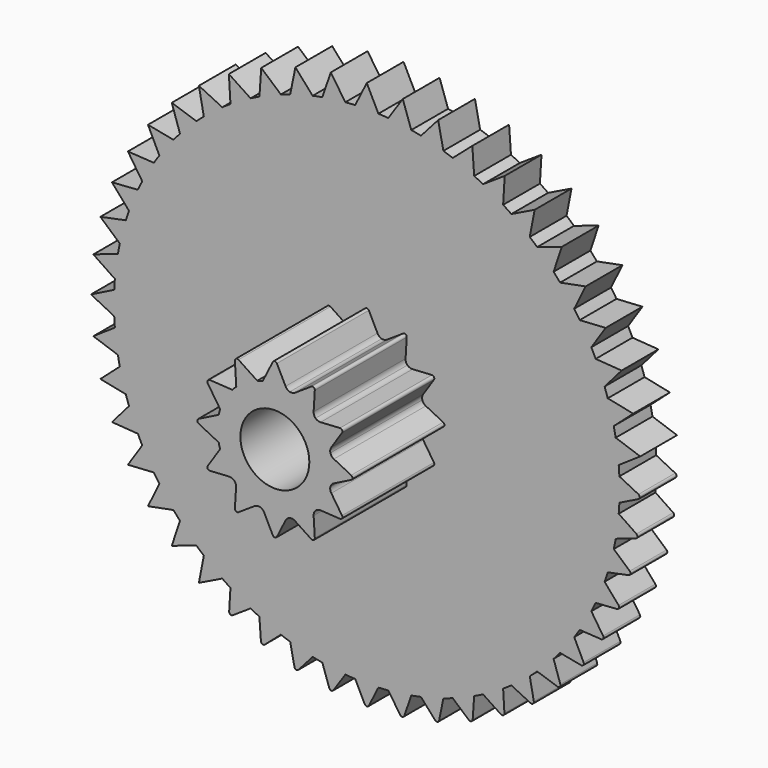
from build123d import *

# Parameters (mm, degrees)
F0_R        = 2.5
F1_DEPTH    = 2
F2_R        = 1.5
F3_DEPTH    = 7
F4_R        = 0.1
F5_T1_DEPTH = 5.3474638977


# Not quite as in the source:
# - a fillet or chamfer that OpenCascade refuses, or shapes differently, is made with other operations: its cross-section is extruded or revolved along the edge and cut away or added


with BuildPart() as f1:
    # F0 (on Front) → F1 (new body)
    with BuildSketch(Plane.XZ):
        with BuildLine():
            ThreePointArc((10.9883894401, -0.5052697435), (10.9970969769, -0.2527015625), (11, 0))
            ThreePointArc((11, 0), (10.9970969769, 0.2527015625), (10.9883894401, 0.5052697435))
            ThreePointArc((10.9883894401, 0.5052697435), (10.9764481556, 0.7194344215), (10.9603331808, 0.9333255414))
            ThreePointArc((10.9603331808, 0.9333255414), (10.9058934751, 1.4357881144), (10.8284313095, 1.9352197231))
            ThreePointArc((10.8284313095, 1.9352197231), (10.7886380844, 2.1459935422), (10.744742582, 2.3559513676))
            ThreePointArc((10.744742582, 2.3559513676), (10.6251840892, 2.8470094961), (10.4831957169, 3.3320575566))
            ThreePointArc((10.4831957169, 3.3320575566), (10.4162314244, 3.5358341183), (10.3453064586, 3.7382662127))
            ThreePointArc((10.3453064586, 3.7382662127), (10.1626748576, 4.209517756), (9.9585897392, 4.6718829615))
            ThreePointArc((9.9585897392, 4.6718829615), (9.8656001569, 4.8651755924), (9.7688592735, 5.0566182864))
            ThreePointArc((9.7688592735, 5.0566182864), (9.5262794416, 5.5), (9.26358953, 5.9317711537))
            ThreePointArc((9.26358953, 5.9317711537), (9.1461657353, 6.1112725632), (9.0252641978, 6.2884502193))
            ThreePointArc((9.0252641978, 6.2884502193), (8.7268867432, 6.6963757191), (8.4100867356, 7.0901650968))
            ThreePointArc((8.4100867356, 7.0901650968), (8.2702378823, 7.2528039661), (8.1272443493, 7.4126850254))
            ThreePointArc((8.1272443493, 7.4126850254), (7.7781745931, 7.7781745931), (7.4126850254, 8.1272443493))
            ThreePointArc((7.4126850254, 8.1272443493), (7.2528039661, 8.2702378823), (7.0901650968, 8.4100867356))
            ThreePointArc((7.0901650968, 8.4100867356), (6.6963757191, 8.7268867432), (6.2884502193, 9.0252641978))
            ThreePointArc((6.2884502193, 9.0252641978), (6.1112725632, 9.1461657353), (5.9317711537, 9.26358953))
            ThreePointArc((5.9317711537, 9.26358953), (5.5, 9.5262794416), (5.0566182864, 9.7688592735))
            ThreePointArc((5.0566182864, 9.7688592735), (4.8651755924, 9.8656001569), (4.6718829615, 9.9585897392))
            ThreePointArc((4.6718829615, 9.9585897392), (4.209517756, 10.1626748576), (3.7382662127, 10.3453064586))
            ThreePointArc((3.7382662127, 10.3453064586), (3.5358341183, 10.4162314244), (3.3320575566, 10.4831957169))
            ThreePointArc((3.3320575566, 10.4831957169), (2.8470094961, 10.6251840892), (2.3559513676, 10.744742582))
            ThreePointArc((2.3559513676, 10.744742582), (2.1459935422, 10.7886380844), (1.9352197231, 10.8284313095))
            ThreePointArc((1.9352197231, 10.8284313095), (1.4357881144, 10.9058934751), (0.9333255414, 10.9603331808))
            ThreePointArc((0.9333255414, 10.9603331808), (0.7194344215, 10.9764481556), (0.5052697435, 10.9883894401))
            ThreePointArc((0.5052697435, 10.9883894401), (0.2527015625, 10.9970969769), (0, 11))
            ThreePointArc((0, 11), (-0.2527015625, 10.9970969769), (-0.5052697435, 10.9883894401))
            ThreePointArc((-0.5052697435, 10.9883894401), (-0.7194344215, 10.9764481556), (-0.9333255414, 10.9603331808))
            ThreePointArc((-0.9333255414, 10.9603331808), (-1.4357881144, 10.9058934751), (-1.9352197231, 10.8284313095))
            ThreePointArc((-1.9352197231, 10.8284313095), (-2.1459935422, 10.7886380844), (-2.3559513676, 10.744742582))
            ThreePointArc((-2.3559513676, 10.744742582), (-2.8470094961, 10.6251840892), (-3.3320575566, 10.4831957169))
            ThreePointArc((-3.3320575566, 10.4831957169), (-3.5358341183, 10.4162314244), (-3.7382662127, 10.3453064586))
            ThreePointArc((-3.7382662127, 10.3453064586), (-4.209517756, 10.1626748576), (-4.6718829615, 9.9585897392))
            ThreePointArc((-4.6718829615, 9.9585897392), (-4.8651755924, 9.8656001569), (-5.0566182864, 9.7688592735))
            ThreePointArc((-5.0566182864, 9.7688592735), (-5.5, 9.5262794416), (-5.9317711537, 9.26358953))
            ThreePointArc((-5.9317711537, 9.26358953), (-6.1112725632, 9.1461657353), (-6.2884502193, 9.0252641978))
            ThreePointArc((-6.2884502193, 9.0252641978), (-6.6963757191, 8.7268867432), (-7.0901650968, 8.4100867356))
            ThreePointArc((-7.0901650968, 8.4100867356), (-7.2528039661, 8.2702378823), (-7.4126850254, 8.1272443493))
            ThreePointArc((-7.4126850254, 8.1272443493), (-7.7781745931, 7.7781745931), (-8.1272443493, 7.4126850254))
            ThreePointArc((-8.1272443493, 7.4126850254), (-8.2702378823, 7.2528039661), (-8.4100867356, 7.0901650968))
            ThreePointArc((-8.4100867356, 7.0901650968), (-8.7268867432, 6.6963757191), (-9.0252641978, 6.2884502193))
            ThreePointArc((-9.0252641978, 6.2884502193), (-9.1461657353, 6.1112725632), (-9.26358953, 5.9317711537))
            ThreePointArc((-9.26358953, 5.9317711537), (-9.5262794416, 5.5), (-9.7688592735, 5.0566182864))
            ThreePointArc((-9.7688592735, 5.0566182864), (-9.8656001569, 4.8651755924), (-9.9585897392, 4.6718829615))
            ThreePointArc((-9.9585897392, 4.6718829615), (-10.1626748576, 4.209517756), (-10.3453064586, 3.7382662127))
            ThreePointArc((-10.3453064586, 3.7382662127), (-10.4162314244, 3.5358341183), (-10.4831957169, 3.3320575566))
            ThreePointArc((-10.4831957169, 3.3320575566), (-10.6251840892, 2.8470094961), (-10.744742582, 2.3559513676))
            ThreePointArc((-10.744742582, 2.3559513676), (-10.7886380844, 2.1459935422), (-10.8284313095, 1.9352197231))
            ThreePointArc((-10.8284313095, 1.9352197231), (-10.9058934751, 1.4357881144), (-10.9603331808, 0.9333255414))
            ThreePointArc((-10.9603331808, 0.9333255414), (-10.9764481556, 0.7194344215), (-10.9883894401, 0.5052697435))
            ThreePointArc((-10.9883894401, 0.5052697435), (-11, 0), (-10.9883894401, -0.5052697435))
            ThreePointArc((-10.9883894401, -0.5052697435), (-10.9764481556, -0.7194344215), (-10.9603331808, -0.9333255414))
            ThreePointArc((-10.9603331808, -0.9333255414), (-10.9058934751, -1.4357881144), (-10.8284313095, -1.9352197231))
            ThreePointArc((-10.8284313095, -1.9352197231), (-10.7886380844, -2.1459935422), (-10.744742582, -2.3559513676))
            ThreePointArc((-10.744742582, -2.3559513676), (-10.6251840892, -2.8470094961), (-10.4831957169, -3.3320575566))
            ThreePointArc((-10.4831957169, -3.3320575566), (-10.4162314244, -3.5358341183), (-10.3453064586, -3.7382662127))
            ThreePointArc((-10.3453064586, -3.7382662127), (-10.1626748576, -4.209517756), (-9.9585897392, -4.6718829615))
            ThreePointArc((-9.9585897392, -4.6718829615), (-9.8656001569, -4.8651755924), (-9.7688592735, -5.0566182864))
            ThreePointArc((-9.7688592735, -5.0566182864), (-9.5262794416, -5.5), (-9.26358953, -5.9317711537))
            ThreePointArc((-9.26358953, -5.9317711537), (-9.1461657353, -6.1112725632), (-9.0252641978, -6.2884502193))
            ThreePointArc((-9.0252641978, -6.2884502193), (-8.7268867432, -6.6963757191), (-8.4100867356, -7.0901650968))
            ThreePointArc((-8.4100867356, -7.0901650968), (-8.2702378823, -7.2528039661), (-8.1272443493, -7.4126850254))
            ThreePointArc((-8.1272443493, -7.4126850254), (-7.7781745931, -7.7781745931), (-7.4126850254, -8.1272443493))
            ThreePointArc((-7.4126850254, -8.1272443493), (-7.2528039661, -8.2702378823), (-7.0901650968, -8.4100867356))
            ThreePointArc((-7.0901650968, -8.4100867356), (-6.6963757191, -8.7268867432), (-6.2884502193, -9.0252641978))
            ThreePointArc((-6.2884502193, -9.0252641978), (-6.1112725632, -9.1461657353), (-5.9317711537, -9.26358953))
            ThreePointArc((-5.9317711537, -9.26358953), (-5.5, -9.5262794416), (-5.0566182864, -9.7688592735))
            ThreePointArc((-5.0566182864, -9.7688592735), (-4.8651755924, -9.8656001569), (-4.6718829615, -9.9585897392))
            ThreePointArc((-4.6718829615, -9.9585897392), (-4.209517756, -10.1626748576), (-3.7382662127, -10.3453064586))
            ThreePointArc((-3.7382662127, -10.3453064586), (-3.5358341183, -10.4162314244), (-3.3320575566, -10.4831957169))
            ThreePointArc((-3.3320575566, -10.4831957169), (-2.8470094961, -10.6251840892), (-2.3559513676, -10.744742582))
            ThreePointArc((-2.3559513676, -10.744742582), (-2.1459935422, -10.7886380844), (-1.9352197231, -10.8284313095))
            ThreePointArc((-1.9352197231, -10.8284313095), (-1.4357881144, -10.9058934751), (-0.9333255414, -10.9603331808))
            ThreePointArc((-0.9333255414, -10.9603331808), (-0.7194344215, -10.9764481556), (-0.5052697435, -10.9883894401))
            ThreePointArc((-0.5052697435, -10.9883894401), (0, -11), (0.5052697435, -10.9883894401))
            ThreePointArc((0.5052697435, -10.9883894401), (0.7194344215, -10.9764481556), (0.9333255414, -10.9603331808))
            ThreePointArc((0.9333255414, -10.9603331808), (1.4357881144, -10.9058934751), (1.9352197231, -10.8284313095))
            ThreePointArc((1.9352197231, -10.8284313095), (2.1459935422, -10.7886380844), (2.3559513676, -10.744742582))
            ThreePointArc((2.3559513676, -10.744742582), (2.8470094961, -10.6251840892), (3.3320575566, -10.4831957169))
            ThreePointArc((3.3320575566, -10.4831957169), (3.5358341183, -10.4162314244), (3.7382662127, -10.3453064586))
            ThreePointArc((3.7382662127, -10.3453064586), (4.209517756, -10.1626748576), (4.6718829615, -9.9585897392))
            ThreePointArc((4.6718829615, -9.9585897392), (4.8651755924, -9.8656001569), (5.0566182864, -9.7688592735))
            ThreePointArc((5.0566182864, -9.7688592735), (5.5, -9.5262794416), (5.9317711537, -9.26358953))
            ThreePointArc((5.9317711537, -9.26358953), (6.1112725632, -9.1461657353), (6.2884502193, -9.0252641978))
            ThreePointArc((6.2884502193, -9.0252641978), (6.6963757191, -8.7268867432), (7.0901650968, -8.4100867356))
            ThreePointArc((7.0901650968, -8.4100867356), (7.2528039661, -8.2702378823), (7.4126850254, -8.1272443493))
            ThreePointArc((7.4126850254, -8.1272443493), (7.7781745931, -7.7781745931), (8.1272443493, -7.4126850254))
            ThreePointArc((8.1272443493, -7.4126850254), (8.2702378823, -7.2528039661), (8.4100867356, -7.0901650968))
            ThreePointArc((8.4100867356, -7.0901650968), (8.7268867432, -6.6963757191), (9.0252641978, -6.2884502193))
            ThreePointArc((9.0252641978, -6.2884502193), (9.1461657353, -6.1112725632), (9.26358953, -5.9317711537))
            ThreePointArc((9.26358953, -5.9317711537), (9.5262794416, -5.5), (9.7688592735, -5.0566182864))
            ThreePointArc((9.7688592735, -5.0566182864), (9.8656001569, -4.8651755924), (9.9585897392, -4.6718829615))
            ThreePointArc((9.9585897392, -4.6718829615), (10.1626748576, -4.209517756), (10.3453064586, -3.7382662127))
            ThreePointArc((10.3453064586, -3.7382662127), (10.4162314244, -3.5358341183), (10.4831957169, -3.3320575566))
            ThreePointArc((10.4831957169, -3.3320575566), (10.6251840892, -2.8470094961), (10.744742582, -2.3559513676))
            ThreePointArc((10.744742582, -2.3559513676), (10.7886380844, -2.1459935422), (10.8284313095, -1.9352197231))
            ThreePointArc((10.8284313095, -1.9352197231), (10.9058934751, -1.4357881144), (10.9603331808, -0.9333255414))
            ThreePointArc((10.9603331808, -0.9333255414), (10.9764481556, -0.7194344215), (10.9883894401, -0.5052697435))
        make_face()
        Circle(F0_R, mode=Mode.SUBTRACT)
        with BuildLine():
            ThreePointArc((10.9883894401, 0.5052697435), (10.9970969769, 0.2527015625), (11, 0))
            ThreePointArc((11, 0), (10.9970969769, -0.2527015625), (10.9883894401, -0.5052697435))
            Line((10.9883894401, -0.5052697435), (12, 0))
            Line((12, 0), (10.9883894401, 0.5052697435))
        make_face()
        with BuildLine():
            ThreePointArc((10.8284313095, 1.9352197231), (10.9058934751, 1.4357881144), (10.9603331808, 0.9333255414))
            Line((10.9603331808, 0.9333255414), (11.8973383365, 1.5663143066))
            Line((11.8973383365, 1.5663143066), (10.8284313095, 1.9352197231))
        make_face()
        with BuildLine():
            Line((11.8973383365, -1.5663143066), (10.9603331808, -0.9333255414))
            ThreePointArc((10.9603331808, -0.9333255414), (10.9058934751, -1.4357881144), (10.8284313095, -1.9352197231))
            Line((10.8284313095, -1.9352197231), (11.8973383365, -1.5663143066))
        make_face()
        with BuildLine():
            ThreePointArc((10.4831957169, 3.3320575566), (10.6251840892, 2.8470094961), (10.744742582, 2.3559513676))
            Line((10.744742582, 2.3559513676), (11.5911099155, 3.1058285412))
            Line((11.5911099155, 3.1058285412), (10.4831957169, 3.3320575566))
        make_face()
        with BuildLine():
            Line((11.5911099155, -3.1058285412), (10.744742582, -2.3559513676))
            ThreePointArc((10.744742582, -2.3559513676), (10.6251840892, -2.8470094961), (10.4831957169, -3.3320575566))
            Line((10.4831957169, -3.3320575566), (11.5911099155, -3.1058285412))
        make_face()
        with BuildLine():
            ThreePointArc((9.9585897392, 4.6718829615), (10.1626748576, 4.209517756), (10.3453064586, 3.7382662127))
            Line((10.3453064586, 3.7382662127), (11.0865543901, 4.5922011884))
            Line((11.0865543901, 4.5922011884), (9.9585897392, 4.6718829615))
        make_face()
        with BuildLine():
            Line((11.0865543901, -4.5922011884), (10.3453064586, -3.7382662127))
            ThreePointArc((10.3453064586, -3.7382662127), (10.1626748576, -4.209517756), (9.9585897392, -4.6718829615))
            Line((9.9585897392, -4.6718829615), (11.0865543901, -4.5922011884))
        make_face()
        with BuildLine():
            ThreePointArc((9.26358953, 5.9317711537), (9.5262794416, 5.5), (9.7688592735, 5.0566182864))
            Line((9.7688592735, 5.0566182864), (10.3923048454, 6))
            Line((10.3923048454, 6), (9.26358953, 5.9317711537))
        make_face()
        with BuildLine():
            Line((10.3923048454, -6), (9.7688592735, -5.0566182864))
            ThreePointArc((9.7688592735, -5.0566182864), (9.5262794416, -5.5), (9.26358953, -5.9317711537))
            Line((9.26358953, -5.9317711537), (10.3923048454, -6))
        make_face()
        with BuildLine():
            ThreePointArc((8.4100867356, 7.0901650968), (8.7268867432, 6.6963757191), (9.0252641978, 6.2884502193))
            Line((9.0252641978, 6.2884502193), (9.5202400835, 7.3051371481))
            Line((9.5202400835, 7.3051371481), (8.4100867356, 7.0901650968))
        make_face()
        with BuildLine():
            Line((9.5202400835, -7.3051371481), (9.0252641978, -6.2884502193))
            ThreePointArc((9.0252641978, -6.2884502193), (8.7268867432, -6.6963757191), (8.4100867356, -7.0901650968))
            Line((8.4100867356, -7.0901650968), (9.5202400835, -7.3051371481))
        make_face()
        with BuildLine():
            ThreePointArc((7.4126850254, 8.1272443493), (7.7781745931, 7.7781745931), (8.1272443493, 7.4126850254))
            Line((8.1272443493, 7.4126850254), (8.4852813742, 8.4852813742))
            Line((8.4852813742, 8.4852813742), (7.4126850254, 8.1272443493))
        make_face()
        with BuildLine():
            Line((8.4852813742, -8.4852813742), (8.1272443493, -7.4126850254))
            ThreePointArc((8.1272443493, -7.4126850254), (7.7781745931, -7.7781745931), (7.4126850254, -8.1272443493))
            Line((7.4126850254, -8.1272443493), (8.4852813742, -8.4852813742))
        make_face()
        with BuildLine():
            ThreePointArc((6.2884502193, 9.0252641978), (6.6963757191, 8.7268867432), (7.0901650968, 8.4100867356))
            Line((7.0901650968, 8.4100867356), (7.3051371481, 9.5202400835))
            Line((7.3051371481, 9.5202400835), (6.2884502193, 9.0252641978))
        make_face()
        with BuildLine():
            Line((7.3051371481, -9.5202400835), (7.0901650968, -8.4100867356))
            ThreePointArc((7.0901650968, -8.4100867356), (6.6963757191, -8.7268867432), (6.2884502193, -9.0252641978))
            Line((6.2884502193, -9.0252641978), (7.3051371481, -9.5202400835))
        make_face()
        with BuildLine():
            ThreePointArc((5.0566182864, 9.7688592735), (5.5, 9.5262794416), (5.9317711537, 9.26358953))
            Line((5.9317711537, 9.26358953), (6, 10.3923048454))
            Line((6, 10.3923048454), (5.0566182864, 9.7688592735))
        make_face()
        with BuildLine():
            Line((6, -10.3923048454), (5.9317711537, -9.26358953))
            ThreePointArc((5.9317711537, -9.26358953), (5.5, -9.5262794416), (5.0566182864, -9.7688592735))
            Line((5.0566182864, -9.7688592735), (6, -10.3923048454))
        make_face()
        with BuildLine():
            ThreePointArc((3.7382662127, 10.3453064586), (4.209517756, 10.1626748576), (4.6718829615, 9.9585897392))
            Line((4.6718829615, 9.9585897392), (4.5922011884, 11.0865543901))
            Line((4.5922011884, 11.0865543901), (3.7382662127, 10.3453064586))
        make_face()
        with BuildLine():
            Line((4.5922011884, -11.0865543901), (4.6718829615, -9.9585897392))
            ThreePointArc((4.6718829615, -9.9585897392), (4.209517756, -10.1626748576), (3.7382662127, -10.3453064586))
            Line((3.7382662127, -10.3453064586), (4.5922011884, -11.0865543901))
        make_face()
        with BuildLine():
            ThreePointArc((2.3559513676, 10.744742582), (2.8470094961, 10.6251840892), (3.3320575566, 10.4831957169))
            Line((3.3320575566, 10.4831957169), (3.1058285412, 11.5911099155))
            Line((3.1058285412, 11.5911099155), (2.3559513676, 10.744742582))
        make_face()
        with BuildLine():
            Line((3.1058285412, -11.5911099155), (3.3320575566, -10.4831957169))
            ThreePointArc((3.3320575566, -10.4831957169), (2.8470094961, -10.6251840892), (2.3559513676, -10.744742582))
            Line((2.3559513676, -10.744742582), (3.1058285412, -11.5911099155))
        make_face()
        with BuildLine():
            ThreePointArc((0.9333255414, 10.9603331808), (1.4357881144, 10.9058934751), (1.9352197231, 10.8284313095))
            Line((1.9352197231, 10.8284313095), (1.5663143066, 11.8973383365))
            Line((1.5663143066, 11.8973383365), (0.9333255414, 10.9603331808))
        make_face()
        with BuildLine():
            Line((1.5663143066, -11.8973383365), (1.9352197231, -10.8284313095))
            ThreePointArc((1.9352197231, -10.8284313095), (1.4357881144, -10.9058934751), (0.9333255414, -10.9603331808))
            Line((0.9333255414, -10.9603331808), (1.5663143066, -11.8973383365))
        make_face()
        with BuildLine():
            ThreePointArc((0, 11), (0.2527015625, 10.9970969769), (0.5052697435, 10.9883894401))
            Line((0.5052697435, 10.9883894401), (0, 12))
            Line((0, 12), (0, 11))
        make_face()
        with BuildLine():
            Line((0, -12), (0.5052697435, -10.9883894401))
            ThreePointArc((0.5052697435, -10.9883894401), (0, -11), (-0.5052697435, -10.9883894401))
            Line((-0.5052697435, -10.9883894401), (0, -12))
        make_face()
        with BuildLine():
            ThreePointArc((-0.5052697435, 10.9883894401), (-0.2527015625, 10.9970969769), (0, 11))
            Line((0, 11), (0, 12))
            Line((0, 12), (-0.5052697435, 10.9883894401))
        make_face()
        with BuildLine():
            Line((-1.5663143066, -11.8973383365), (-0.9333255414, -10.9603331808))
            ThreePointArc((-0.9333255414, -10.9603331808), (-1.4357881144, -10.9058934751), (-1.9352197231, -10.8284313095))
            Line((-1.9352197231, -10.8284313095), (-1.5663143066, -11.8973383365))
        make_face()
        with BuildLine():
            ThreePointArc((-1.9352197231, 10.8284313095), (-1.4357881144, 10.9058934751), (-0.9333255414, 10.9603331808))
            Line((-0.9333255414, 10.9603331808), (-1.5663143066, 11.8973383365))
            Line((-1.5663143066, 11.8973383365), (-1.9352197231, 10.8284313095))
        make_face()
        with BuildLine():
            Line((-3.1058285412, -11.5911099155), (-2.3559513676, -10.744742582))
            ThreePointArc((-2.3559513676, -10.744742582), (-2.8470094961, -10.6251840892), (-3.3320575566, -10.4831957169))
            Line((-3.3320575566, -10.4831957169), (-3.1058285412, -11.5911099155))
        make_face()
        with BuildLine():
            ThreePointArc((-3.3320575566, 10.4831957169), (-2.8470094961, 10.6251840892), (-2.3559513676, 10.744742582))
            Line((-2.3559513676, 10.744742582), (-3.1058285412, 11.5911099155))
            Line((-3.1058285412, 11.5911099155), (-3.3320575566, 10.4831957169))
        make_face()
        with BuildLine():
            Line((-4.5922011884, -11.0865543901), (-3.7382662127, -10.3453064586))
            ThreePointArc((-3.7382662127, -10.3453064586), (-4.209517756, -10.1626748576), (-4.6718829615, -9.9585897392))
            Line((-4.6718829615, -9.9585897392), (-4.5922011884, -11.0865543901))
        make_face()
        with BuildLine():
            ThreePointArc((-4.6718829615, 9.9585897392), (-4.209517756, 10.1626748576), (-3.7382662127, 10.3453064586))
            Line((-3.7382662127, 10.3453064586), (-4.5922011884, 11.0865543901))
            Line((-4.5922011884, 11.0865543901), (-4.6718829615, 9.9585897392))
        make_face()
        with BuildLine():
            Line((-6, -10.3923048454), (-5.0566182864, -9.7688592735))
            ThreePointArc((-5.0566182864, -9.7688592735), (-5.5, -9.5262794416), (-5.9317711537, -9.26358953))
            Line((-5.9317711537, -9.26358953), (-6, -10.3923048454))
        make_face()
        with BuildLine():
            ThreePointArc((-5.9317711537, 9.26358953), (-5.5, 9.5262794416), (-5.0566182864, 9.7688592735))
            Line((-5.0566182864, 9.7688592735), (-6, 10.3923048454))
            Line((-6, 10.3923048454), (-5.9317711537, 9.26358953))
        make_face()
        with BuildLine():
            Line((-7.3051371481, -9.5202400835), (-6.2884502193, -9.0252641978))
            ThreePointArc((-6.2884502193, -9.0252641978), (-6.6963757191, -8.7268867432), (-7.0901650968, -8.4100867356))
            Line((-7.0901650968, -8.4100867356), (-7.3051371481, -9.5202400835))
        make_face()
        with BuildLine():
            ThreePointArc((-7.0901650968, 8.4100867356), (-6.6963757191, 8.7268867432), (-6.2884502193, 9.0252641978))
            Line((-6.2884502193, 9.0252641978), (-7.3051371481, 9.5202400835))
            Line((-7.3051371481, 9.5202400835), (-7.0901650968, 8.4100867356))
        make_face()
        with BuildLine():
            Line((-8.4852813742, -8.4852813742), (-7.4126850254, -8.1272443493))
            ThreePointArc((-7.4126850254, -8.1272443493), (-7.7781745931, -7.7781745931), (-8.1272443493, -7.4126850254))
            Line((-8.1272443493, -7.4126850254), (-8.4852813742, -8.4852813742))
        make_face()
        with BuildLine():
            ThreePointArc((-8.1272443493, 7.4126850254), (-7.7781745931, 7.7781745931), (-7.4126850254, 8.1272443493))
            Line((-7.4126850254, 8.1272443493), (-8.4852813742, 8.4852813742))
            Line((-8.4852813742, 8.4852813742), (-8.1272443493, 7.4126850254))
        make_face()
        with BuildLine():
            Line((-9.5202400835, -7.3051371481), (-8.4100867356, -7.0901650968))
            ThreePointArc((-8.4100867356, -7.0901650968), (-8.7268867432, -6.6963757191), (-9.0252641978, -6.2884502193))
            Line((-9.0252641978, -6.2884502193), (-9.5202400835, -7.3051371481))
        make_face()
        with BuildLine():
            ThreePointArc((-9.0252641978, 6.2884502193), (-8.7268867432, 6.6963757191), (-8.4100867356, 7.0901650968))
            Line((-8.4100867356, 7.0901650968), (-9.5202400835, 7.3051371481))
            Line((-9.5202400835, 7.3051371481), (-9.0252641978, 6.2884502193))
        make_face()
        with BuildLine():
            Line((-10.3923048454, -6), (-9.26358953, -5.9317711537))
            ThreePointArc((-9.26358953, -5.9317711537), (-9.5262794416, -5.5), (-9.7688592735, -5.0566182864))
            Line((-9.7688592735, -5.0566182864), (-10.3923048454, -6))
        make_face()
        with BuildLine():
            ThreePointArc((-9.7688592735, 5.0566182864), (-9.5262794416, 5.5), (-9.26358953, 5.9317711537))
            Line((-9.26358953, 5.9317711537), (-10.3923048454, 6))
            Line((-10.3923048454, 6), (-9.7688592735, 5.0566182864))
        make_face()
        with BuildLine():
            Line((-11.0865543901, -4.5922011884), (-9.9585897392, -4.6718829615))
            ThreePointArc((-9.9585897392, -4.6718829615), (-10.1626748576, -4.209517756), (-10.3453064586, -3.7382662127))
            Line((-10.3453064586, -3.7382662127), (-11.0865543901, -4.5922011884))
        make_face()
        with BuildLine():
            ThreePointArc((-10.3453064586, 3.7382662127), (-10.1626748576, 4.209517756), (-9.9585897392, 4.6718829615))
            Line((-9.9585897392, 4.6718829615), (-11.0865543901, 4.5922011884))
            Line((-11.0865543901, 4.5922011884), (-10.3453064586, 3.7382662127))
        make_face()
        with BuildLine():
            Line((-11.5911099155, -3.1058285412), (-10.4831957169, -3.3320575566))
            ThreePointArc((-10.4831957169, -3.3320575566), (-10.6251840892, -2.8470094961), (-10.744742582, -2.3559513676))
            Line((-10.744742582, -2.3559513676), (-11.5911099155, -3.1058285412))
        make_face()
        with BuildLine():
            ThreePointArc((-10.744742582, 2.3559513676), (-10.6251840892, 2.8470094961), (-10.4831957169, 3.3320575566))
            Line((-10.4831957169, 3.3320575566), (-11.5911099155, 3.1058285412))
            Line((-11.5911099155, 3.1058285412), (-10.744742582, 2.3559513676))
        make_face()
        with BuildLine():
            Line((-11.8973383365, -1.5663143066), (-10.8284313095, -1.9352197231))
            ThreePointArc((-10.8284313095, -1.9352197231), (-10.9058934751, -1.4357881144), (-10.9603331808, -0.9333255414))
            Line((-10.9603331808, -0.9333255414), (-11.8973383365, -1.5663143066))
        make_face()
        with BuildLine():
            ThreePointArc((-10.9603331808, 0.9333255414), (-10.9058934751, 1.4357881144), (-10.8284313095, 1.9352197231))
            Line((-10.8284313095, 1.9352197231), (-11.8973383365, 1.5663143066))
            Line((-11.8973383365, 1.5663143066), (-10.9603331808, 0.9333255414))
        make_face()
        with BuildLine():
            Line((-12, 0), (-10.9883894401, -0.5052697435))
            ThreePointArc((-10.9883894401, -0.5052697435), (-11, 0), (-10.9883894401, 0.5052697435))
            Line((-10.9883894401, 0.5052697435), (-12, 0))
        make_face()
    extrude(amount=F1_DEPTH)

    # F2 (on Front) → F3 (join)
    with BuildSketch(Plane.XZ):
        with BuildLine():
            ThreePointArc((2.4436492953, -0.5278050033), (2.485872406, -0.2654023), (2.5, 0))
            ThreePointArc((2.5, 0), (2.485872406, 0.2654023), (2.4436492953, 0.5278050033))
            ThreePointArc((2.4436492953, 0.5278050033), (2.4148145657, 0.6470476128), (2.3801648693, 0.7647321065))
            ThreePointArc((2.3801648693, 0.7647321065), (2.1650635095, 1.25), (1.852359866, 1.6789171888))
            ThreePointArc((1.852359866, 1.6789171888), (1.767766953, 1.767766953), (1.6789171888, 1.852359866))
            ThreePointArc((1.6789171888, 1.852359866), (1.25, 2.1650635095), (0.7647321065, 2.3801648693))
            ThreePointArc((0.7647321065, 2.3801648693), (0.6470476128, 2.4148145657), (0.5278050033, 2.4436492953))
            ThreePointArc((0.5278050033, 2.4436492953), (0.2654023, 2.485872406), (0, 2.5))
            ThreePointArc((0, 2.5), (-0.2654023, 2.485872406), (-0.5278050033, 2.4436492953))
            ThreePointArc((-0.5278050033, 2.4436492953), (-0.6470476128, 2.4148145657), (-0.7647321065, 2.3801648693))
            ThreePointArc((-0.7647321065, 2.3801648693), (-1.25, 2.1650635095), (-1.6789171888, 1.852359866))
            ThreePointArc((-1.6789171888, 1.852359866), (-1.767766953, 1.767766953), (-1.852359866, 1.6789171888))
            ThreePointArc((-1.852359866, 1.6789171888), (-2.1650635095, 1.25), (-2.3801648693, 0.7647321065))
            ThreePointArc((-2.3801648693, 0.7647321065), (-2.4148145657, 0.6470476128), (-2.4436492953, 0.5278050033))
            ThreePointArc((-2.4436492953, 0.5278050033), (-2.5, 0), (-2.4436492953, -0.5278050033))
            ThreePointArc((-2.4436492953, -0.5278050033), (-2.4148145657, -0.6470476128), (-2.3801648693, -0.7647321065))
            ThreePointArc((-2.3801648693, -0.7647321065), (-2.1650635095, -1.25), (-1.852359866, -1.6789171888))
            ThreePointArc((-1.852359866, -1.6789171888), (-1.767766953, -1.767766953), (-1.6789171888, -1.852359866))
            ThreePointArc((-1.6789171888, -1.852359866), (-1.25, -2.1650635095), (-0.7647321065, -2.3801648693))
            ThreePointArc((-0.7647321065, -2.3801648693), (-0.6470476128, -2.4148145657), (-0.5278050033, -2.4436492953))
            ThreePointArc((-0.5278050033, -2.4436492953), (0, -2.5), (0.5278050033, -2.4436492953))
            ThreePointArc((0.5278050033, -2.4436492953), (0.6470476128, -2.4148145657), (0.7647321065, -2.3801648693))
            ThreePointArc((0.7647321065, -2.3801648693), (1.25, -2.1650635095), (1.6789171888, -1.852359866))
            ThreePointArc((1.6789171888, -1.852359866), (1.767766953, -1.767766953), (1.852359866, -1.6789171888))
            ThreePointArc((1.852359866, -1.6789171888), (2.1650635095, -1.25), (2.3801648693, -0.7647321065))
            ThreePointArc((2.3801648693, -0.7647321065), (2.4148145657, -0.6470476128), (2.4436492953, -0.5278050033))
        make_face()
        Circle(F2_R, mode=Mode.SUBTRACT)
        with BuildLine():
            ThreePointArc((2.4436492953, 0.5278050033), (2.485872406, 0.2654023), (2.5, 0))
            ThreePointArc((2.5, 0), (2.485872406, -0.2654023), (2.4436492953, -0.5278050033))
            Line((2.4436492953, -0.5278050033), (3.5, 0))
            Line((3.5, 0), (2.4436492953, 0.5278050033))
        make_face()
        with BuildLine():
            ThreePointArc((1.852359866, 1.6789171888), (2.1650635095, 1.25), (2.3801648693, 0.7647321065))
            Line((2.3801648693, 0.7647321065), (3.0310889132, 1.75))
            Line((3.0310889132, 1.75), (1.852359866, 1.6789171888))
        make_face()
        with BuildLine():
            Line((3.0310889132, -1.75), (2.3801648693, -0.7647321065))
            ThreePointArc((2.3801648693, -0.7647321065), (2.1650635095, -1.25), (1.852359866, -1.6789171888))
            Line((1.852359866, -1.6789171888), (3.0310889132, -1.75))
        make_face()
        with BuildLine():
            ThreePointArc((0.7647321065, 2.3801648693), (1.25, 2.1650635095), (1.6789171888, 1.852359866))
            Line((1.6789171888, 1.852359866), (1.75, 3.0310889132))
            Line((1.75, 3.0310889132), (0.7647321065, 2.3801648693))
        make_face()
        with BuildLine():
            Line((1.75, -3.0310889132), (1.6789171888, -1.852359866))
            ThreePointArc((1.6789171888, -1.852359866), (1.25, -2.1650635095), (0.7647321065, -2.3801648693))
            Line((0.7647321065, -2.3801648693), (1.75, -3.0310889132))
        make_face()
        with BuildLine():
            ThreePointArc((0, 2.5), (0.2654023, 2.485872406), (0.5278050033, 2.4436492953))
            Line((0.5278050033, 2.4436492953), (0.4996494071, 2.5))
            Line((0.4996494071, 2.5), (0, 2.5))
        make_face()
        with BuildLine():
            Line((0, -3.5), (0.5278050033, -2.4436492953))
            ThreePointArc((0.5278050033, -2.4436492953), (0, -2.5), (-0.5278050033, -2.4436492953))
            Line((-0.5278050033, -2.4436492953), (0, -3.5))
        make_face()
        with BuildLine():
            ThreePointArc((-0.5278050033, 2.4436492953), (-0.2654023, 2.485872406), (0, 2.5))
            Line((0, 2.5), (0, 3.5))
            Line((0, 3.5), (-0.5278050033, 2.4436492953))
        make_face()
        Polygon((0, 3.5), (0, 2.5), (0.4996494071, 2.5), align=None)
        with BuildLine():
            Line((-1.75, -3.0310889132), (-0.7647321065, -2.3801648693))
            ThreePointArc((-0.7647321065, -2.3801648693), (-1.25, -2.1650635095), (-1.6789171888, -1.852359866))
            Line((-1.6789171888, -1.852359866), (-1.75, -3.0310889132))
        make_face()
        with BuildLine():
            ThreePointArc((-1.6789171888, 1.852359866), (-1.25, 2.1650635095), (-0.7647321065, 2.3801648693))
            Line((-0.7647321065, 2.3801648693), (-1.75, 3.0310889132))
            Line((-1.75, 3.0310889132), (-1.6789171888, 1.852359866))
        make_face()
        with BuildLine():
            Line((-3.0310889132, -1.75), (-1.852359866, -1.6789171888))
            ThreePointArc((-1.852359866, -1.6789171888), (-2.1650635095, -1.25), (-2.3801648693, -0.7647321065))
            Line((-2.3801648693, -0.7647321065), (-3.0310889132, -1.75))
        make_face()
        with BuildLine():
            ThreePointArc((-2.3801648693, 0.7647321065), (-2.1650635095, 1.25), (-1.852359866, 1.6789171888))
            Line((-1.852359866, 1.6789171888), (-3.0310889132, 1.75))
            Line((-3.0310889132, 1.75), (-2.3801648693, 0.7647321065))
        make_face()
        with BuildLine():
            Line((-3.5, 0), (-2.4436492953, -0.5278050033))
            ThreePointArc((-2.4436492953, -0.5278050033), (-2.5, 0), (-2.4436492953, 0.5278050033))
            Line((-2.4436492953, 0.5278050033), (-3.5, 0))
        make_face()
    extrude(amount=F3_DEPTH)

    # F4
    f4_edges = [f1.edges().sort_by_distance(p)[0] for p in [
        (1.75, -4.5, 3.031089),
        (3.031089, -4.5, 1.75),
        (3.5, -4.5, 0),
        (3.031089, -4.5, -1.75),
        (1.75, -4.5, -3.031089),
        (0, -4.5, -3.5),
        (-1.75, -4.5, -3.031089),
        (-3.031089, -4.5, -1.75),
        (-3.5, -4.5, 0),
        (-3.031089, -4.5, 1.75),
        (-1.75, -4.5, 3.031089),
        (0, -4.5, 3.5),
        (-6, -1, -10.392305),
        (-4.592201, -1, -11.086554),
        (-3.105829, -1, -11.59111),
        (-1.566314, -1, -11.897338),
        (0, -1, -12),
        (1.566314, -1, -11.897338),
        (3.105829, -1, -11.59111),
        (4.592201, -1, -11.086554),
        (6, -1, -10.392305),
        (7.305137, -1, -9.52024),
        (8.485281, -1, -8.485281),
        (9.52024, -1, -7.305137),
        (10.392305, -1, -6),
        (11.086554, -1, -4.592201),
        (11.59111, -1, -3.105829),
        (11.897338, -1, -1.566314),
        (12, -1, 0),
    ]]
    fillet(f4_edges, radius=F4_R)

    # F5: fillet of radius 0.3 on 16 edges, made by hand

    # F5_s2 → F5_t1 (join)
    with BuildSketch(Plane.XZ.offset(1.6525361023)):
        with BuildLine():
            ThreePointArc((0.6554012742, 2.412560708), (0.5439352673, 2.4699977315), (0.4656836455, 2.5679791893))
            Line((0.4656836455, 2.5679791893), (0.5278050033, 2.4436492953))
            ThreePointArc((0.5278050033, 2.4436492953), (0.5918073156, 2.4289430008), (0.6554012742, 2.412560708))
        make_face()
        with BuildLine():
            ThreePointArc((0.8806957275, 2.4567770371), (0.7639371063, 2.4110484164), (0.6386862009, 2.4170394984))
            ThreePointArc((0.6386862009, 2.4170394984), (0.7019513309, 2.3994300009), (0.7647321065, 2.3801648693))
            Line((0.7647321065, 2.3801648693), (0.8806957275, 2.4567770371))
        make_face()
        with BuildLine():
            ThreePointArc((1.7738745071, 1.7616382242), (1.7060606252, 1.8671131492), (1.6872834618, 1.9910933916))
            Line((1.6872834618, 1.9910933916), (1.6789171888, 1.852359866))
            ThreePointArc((1.6789171888, 1.852359866), (1.7269916699, 1.8076226852), (1.7738745071, 1.7616382242))
        make_face()
        with BuildLine():
            ThreePointArc((1.9910933916, 1.6872834618), (1.8671131492, 1.7060606252), (1.7616382242, 1.7738745071))
            ThreePointArc((1.7616382242, 1.7738745071), (1.8076226852, 1.7269916699), (1.852359866, 1.6789171888))
            Line((1.852359866, 1.6789171888), (1.9910933916, 1.6872834618))
        make_face()
        with BuildLine():
            ThreePointArc((2.4567770371, 0.8806957275), (2.4110484164, 0.7639371063), (2.4170394984, 0.6386862009))
            ThreePointArc((2.4170394984, 0.6386862009), (2.3994300009, 0.7019513309), (2.3801648693, 0.7647321065))
            Line((2.3801648693, 0.7647321065), (2.4567770371, 0.8806957275))
        make_face()
        with BuildLine():
            ThreePointArc((2.412560708, 0.6554012742), (2.4699977315, 0.5439352673), (2.5679791893, 0.4656836455))
            Line((2.5679791893, 0.4656836455), (2.4436492953, 0.5278050033))
            ThreePointArc((2.4436492953, 0.5278050033), (2.4289430008, 0.5918073156), (2.412560708, 0.6554012742))
        make_face()
        with BuildLine():
            ThreePointArc((2.5679791893, -0.4656836455), (2.4699977315, -0.5439352673), (2.412560708, -0.6554012742))
            ThreePointArc((2.412560708, -0.6554012742), (2.4289430008, -0.5918073156), (2.4436492953, -0.5278050033))
            Line((2.4436492953, -0.5278050033), (2.5679791893, -0.4656836455))
        make_face()
        with BuildLine():
            ThreePointArc((2.4170394984, -0.6386862009), (2.4110484164, -0.7639371063), (2.4567770371, -0.8806957275))
            Line((2.4567770371, -0.8806957275), (2.3801648693, -0.7647321065))
            ThreePointArc((2.3801648693, -0.7647321065), (2.3994300009, -0.7019513309), (2.4170394984, -0.6386862009))
        make_face()
        with BuildLine():
            ThreePointArc((1.9910933916, -1.6872834618), (1.8671131492, -1.7060606252), (1.7616382242, -1.7738745071))
            ThreePointArc((1.7616382242, -1.7738745071), (1.8076226852, -1.7269916699), (1.852359866, -1.6789171888))
            Line((1.852359866, -1.6789171888), (1.9910933916, -1.6872834618))
        make_face()
        with BuildLine():
            ThreePointArc((1.7738745071, -1.7616382242), (1.7060606252, -1.8671131492), (1.6872834618, -1.9910933916))
            Line((1.6872834618, -1.9910933916), (1.6789171888, -1.852359866))
            ThreePointArc((1.6789171888, -1.852359866), (1.7269916699, -1.8076226852), (1.7738745071, -1.7616382242))
        make_face()
        with BuildLine():
            ThreePointArc((0.8806957275, -2.4567770371), (0.7639371063, -2.4110484164), (0.6386862009, -2.4170394984))
            ThreePointArc((0.6386862009, -2.4170394984), (0.7019513309, -2.3994300009), (0.7647321065, -2.3801648693))
            Line((0.7647321065, -2.3801648693), (0.8806957275, -2.4567770371))
        make_face()
        with BuildLine():
            ThreePointArc((0.6554012742, -2.412560708), (0.5439352673, -2.4699977315), (0.4656836455, -2.5679791893))
            Line((0.4656836455, -2.5679791893), (0.5278050033, -2.4436492953))
            ThreePointArc((0.5278050033, -2.4436492953), (0.5918073156, -2.4289430008), (0.6554012742, -2.412560708))
        make_face()
        with BuildLine():
            ThreePointArc((-0.4656836455, -2.5679791893), (-0.5439352673, -2.4699977315), (-0.6554012742, -2.412560708))
            ThreePointArc((-0.6554012742, -2.412560708), (-0.5918073156, -2.4289430008), (-0.5278050033, -2.4436492953))
            Line((-0.5278050033, -2.4436492953), (-0.4656836455, -2.5679791893))
        make_face()
        with BuildLine():
            ThreePointArc((-0.6386862009, -2.4170394984), (-0.7639371063, -2.4110484164), (-0.8806957275, -2.4567770371))
            Line((-0.8806957275, -2.4567770371), (-0.7647321065, -2.3801648693))
            ThreePointArc((-0.7647321065, -2.3801648693), (-0.7019513309, -2.3994300009), (-0.6386862009, -2.4170394984))
        make_face()
        with BuildLine():
            ThreePointArc((-1.6872834618, -1.9910933916), (-1.7060606252, -1.8671131492), (-1.7738745071, -1.7616382242))
            ThreePointArc((-1.7738745071, -1.7616382242), (-1.7269916699, -1.8076226852), (-1.6789171888, -1.852359866))
            Line((-1.6789171888, -1.852359866), (-1.6872834618, -1.9910933916))
        make_face()
        with BuildLine():
            ThreePointArc((-1.7616382242, -1.7738745071), (-1.8671131492, -1.7060606252), (-1.9910933916, -1.6872834618))
            Line((-1.9910933916, -1.6872834618), (-1.852359866, -1.6789171888))
            ThreePointArc((-1.852359866, -1.6789171888), (-1.8076226852, -1.7269916699), (-1.7616382242, -1.7738745071))
        make_face()
    extrude(amount=F5_T1_DEPTH)


solid = f1.part
